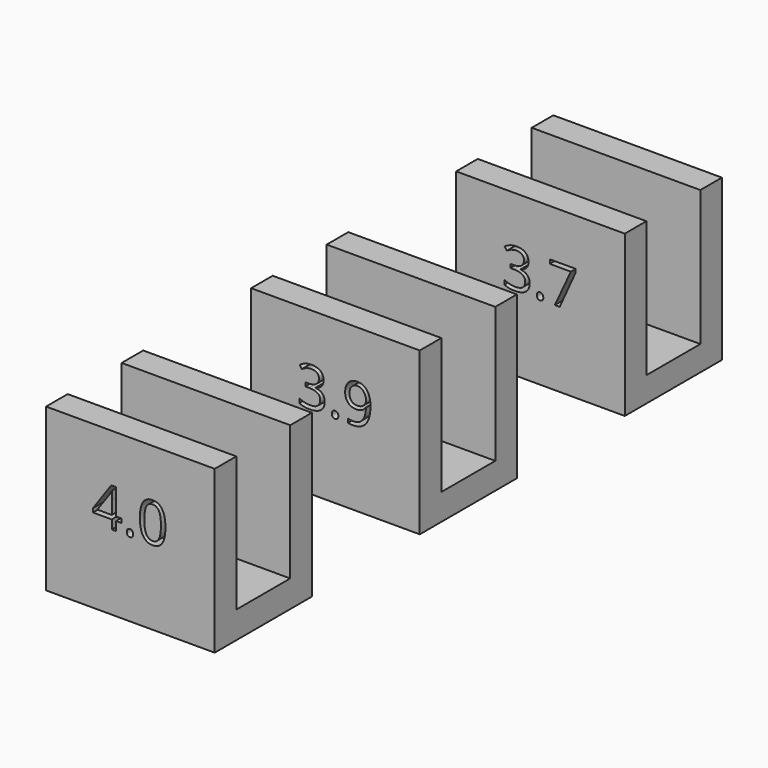
from build123d import *

# Parameters (mm, degrees)
F1_DEPTH     = 25
F2_TEXT_SIZE = 8.0253423502
F5_DEPTH     = 4
F3_TEXT_SIZE = 8.0474069668
F6_DEPTH     = 4
F4_TEXT_SIZE = 8.0315082372
F7_DEPTH     = 4


# Not quite as in the source:
# - Text() gives the source's letters only with a copy of the font that has no kerning and outlines rounded to 1/6400 em; it was checked with that copy


with BuildPart() as f1:
    # F0 (on Right) → F1 (new body)
    with BuildSketch(Plane.YZ):
        Polygon((-47, 0), (-38, 0), (-38, 24), (-42, 24), (-42, 4), (-47, 4), (-52, 4), (-52, 24), (-56, 24), (-56, 0), align=None)
    extrude(amount=F1_DEPTH)

    # F2 (on face) → F5 (cut, through all)
    with BuildSketch(Plane.XZ.offset(56)):
        with Locations((6.7831975352, 11.1108767539)):
            Text('4.0', F2_TEXT_SIZE, font='Open Sans', text_align=(TextAlign.LEFT, TextAlign.BOTTOM))
    extrude(amount=-F5_DEPTH, mode=Mode.SUBTRACT)


with BuildPart() as f1b:
    # F0 (on Right) → F1, piece 2 (new body)
    with BuildSketch(Plane.YZ):
        Polygon((-4, 3.9), (-9, 3.9), (-14, 3.9), (-14, 24), (-18, 24), (-18, 0), (-9, 0), (0, 0), (0, 24), (-4, 24), align=None)
    extrude(amount=F1_DEPTH)

    # F3 (on face) → F6 (cut, through all)
    with BuildSketch(Plane.XZ.offset(18)):
        with Locations((6.7831975352, 11.09499023)):
            Text('3.9', F3_TEXT_SIZE, font='Open Sans', text_align=(TextAlign.LEFT, TextAlign.BOTTOM))
    extrude(amount=-F6_DEPTH, mode=Mode.SUBTRACT)


with BuildPart() as f1c:
    # F0 (on Right) → F1, piece 3 (new body)
    with BuildSketch(Plane.YZ):
        Polygon((20, 0), (29, 0), (38, 0), (38, 23.8), (34, 23.8), (34, 3.7), (29, 3.7), (24, 3.7), (24, 23.8), (20, 23.8), align=None)
    extrude(amount=F1_DEPTH)

    # F4 (on face) → F7 (cut, through all)
    with BuildSketch(Plane.XZ.offset(-20)):
        with Locations((6.7831975352, 11.1064373153)):
            Text('3.7', F4_TEXT_SIZE, font='Open Sans', text_align=(TextAlign.LEFT, TextAlign.BOTTOM))
    extrude(amount=-F7_DEPTH, mode=Mode.SUBTRACT)


solid = Compound([f1.part, f1b.part, f1c.part])
